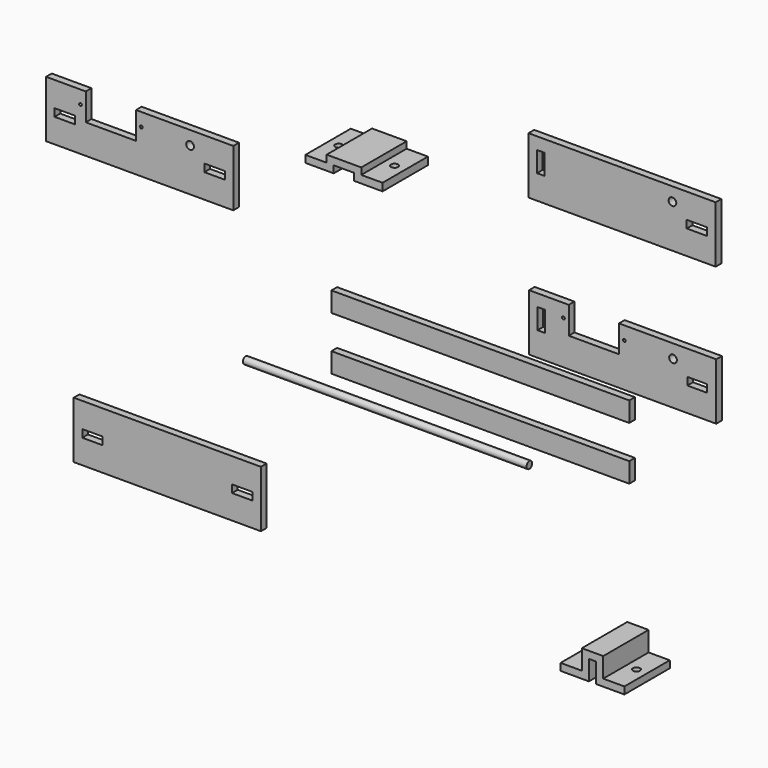
from build123d import *

# Parameters (mm, degrees)
F0_W      = 133.35
F0_H      = 8.89
F1_DEPTH  = 3.175
F2_DEPTH  = 3.175
F0_W_2    = 5.715
F0_H_2    = 3.429
F0_W_3    = 3.429
F0_H_3    = 5.715
F3_DEPTH  = 3.175
F0_W_4    = 8.89
F0_W_5    = 5.461
F4_DEPTH  = 3.175
F5_DEPTH  = 25.4
F6_R      = 1.5875
F8_DEPTH  = 97.2919927368
F0_W_6    = 9.144
F0_R      = 0.635
F0_R_2    = 1.7145
F9_DEPTH  = 3.175
F10_DEPTH = 3.175
F11_R     = 1.5875
F12_DEPTH = 127
F13_DEPTH = 25.4
F16_DEPTH = 6.5659173141


# Not quite as in the source:
# - a feature names something its author has since deleted; it is built from what else it names


with BuildPart() as f1:
    # F0 (on Front) → F1 (new body)
    with BuildSketch(Plane.XZ):
        with Locations((-66.3894339323, -18.7695804912)):
            Rectangle(F0_W, F0_H)
    extrude(amount=F1_DEPTH)


with BuildPart() as f2:
    # F0 (on Front) → F2 (new body)
    with BuildSketch(Plane.XZ):
        with Locations((-66.3894339323, -42.7141800451)):
            Rectangle(F0_W, F0_H)
    extrude(amount=F2_DEPTH)


with BuildPart() as f3:
    # F0 (on Front) → F3 (new body)
    with BuildSketch(Plane.XZ):
        Polygon((-41.0302151682, 76.3552769363), (-44.8402151682, 76.3552769363), (-44.8402151682, 50.9552769363), (38.9797848318, 50.9552769363), (38.9797848318, 76.3552769363), (35.1697848318, 76.3552769363), (19.6249848318, 76.3552769363), (9.5919848318, 76.3552769363), align=None)
        Polygon((-41.0302151682, 65.2427769363), (-41.0302151682, 70.9577769363), (-37.6012151682, 70.9577769363), (-37.6012151682, 65.2427769363), (-31.8862151682, 65.2427769363), (-31.8862151682, 61.8137769363), (-37.6012151682, 61.8137769363), (-41.0302151682, 61.8137769363), align=None, mode=Mode.SUBTRACT)
        with BuildLine():
            ThreePointArc((21.3394848318, 70.2846769363), (18.4126502554, 69.0723423599), (19.6249848318, 71.9991769363))
            ThreePointArc((19.6249848318, 71.9991769363), (20.8373194081, 71.4970115126), (21.3394848318, 70.2846769363))
        make_face(mode=Mode.SUBTRACT)
        Polygon((31.7407848318, 70.9577769363), (35.1697848318, 70.9577769363), (35.1697848318, 65.2427769363), (35.1697848318, 61.8137769363), (31.7407848318, 61.8137769363), (26.0257848318, 61.8137769363), (26.0257848318, 65.2427769363), (31.7407848318, 65.2427769363), align=None, mode=Mode.SUBTRACT)
        with Locations((-34.7437151682, 63.5282769363)):
            Rectangle(F0_W_2, F0_H_2)
        with Locations((33.4552848318, 68.1002769363)):
            Rectangle(F0_W_3, F0_H_3)
    extrude(amount=F3_DEPTH)


with BuildPart() as f4:
    # F0 (on Front) → F4 (new body)
    with BuildSketch(Plane.XZ):
        with BuildLine():
            Line((-40.7762151682, 14.5415), (-44.5862151682, 14.5415))
            Line((-44.5862151682, 14.5415), (-44.5862151682, -10.8585))
            Line((-44.5862151682, -10.8585), (-28.4685809165, -10.8585))
            Line((-28.4685809165, -10.8585), (-5.4275859147, -10.8585))
            Line((-5.4275859147, -10.8585), (35.4237848318, -10.8585))
            Line((35.4237848318, -10.8585), (39.2337848318, -10.8585))
            Line((39.2337848318, -10.8585), (39.2337848318, 14.5415))
            Line((39.2337848318, 14.5415), (9.8332848318, 14.5415))
            Line((9.8332848318, 14.5415), (-1.9396151682, 14.5415))
            Line((-1.9396151682, 14.5415), (-1.9396151682, 9.223375))
            ThreePointArc((-1.9396151682, 9.223375), (-1.4906023622, 9.0373878061), (-1.3046151682, 8.588375))
            ThreePointArc((-1.3046151682, 8.588375), (-1.3079957034, 8.5229391406), (-1.3181013153, 8.4582))
            ThreePointArc((-1.3181013153, 8.4582), (-1.9396151682, 7.953375), (-2.5611290212, 8.4582))
            Line((-2.5611290212, 8.4582), (-4.3272151682, 8.4582))
            Line((-4.3272151682, 8.4582), (-4.3272151682, 2.3749))
            Line((-4.3272151682, 2.3749), (-26.8062151682, 2.3749))
            Line((-26.8062151682, 2.3749), (-26.8062151682, 8.5979))
            Line((-26.8062151682, 8.5979), (-28.5524651682, 8.5979))
            ThreePointArc((-28.5524651682, 8.5979), (-29.6364779743, 8.1488871939), (-29.1874651682, 9.2329))
            Line((-29.1874651682, 9.2329), (-29.1874651682, 14.5415))
            Line((-29.1874651682, 14.5415), (-40.7762151682, 14.5415))
        make_face()
        Polygon((-40.7762151682, 3.429), (-40.7762151682, 9.144), (-37.3472151682, 9.144), (-37.3472151682, 3.429), (-31.8862151682, 3.429), (-31.8862151682, 0), (-37.3472151682, 0), (-40.7762151682, 0), align=None, mode=Mode.SUBTRACT)
        with Locations((30.7247848318, 1.7145)):
            Rectangle(F0_W_4, F0_H_2, mode=Mode.SUBTRACT)
        with BuildLine():
            ThreePointArc((21.5934848318, 8.4582), (19.8789848318, 6.7437), (18.1644848318, 8.4582))
            ThreePointArc((18.1644848318, 8.4582), (19.8789848318, 10.1727), (21.5934848318, 8.4582))
        make_face(mode=Mode.SUBTRACT)
        with BuildLine():
            Line((-26.8062151682, 14.5415), (-29.1874651682, 14.5415))
            Line((-29.1874651682, 14.5415), (-29.1874651682, 9.2329))
            ThreePointArc((-29.1874651682, 9.2329), (-28.7384523622, 9.0469128061), (-28.5524651682, 8.5979))
            Line((-28.5524651682, 8.5979), (-26.8062151682, 8.5979))
            Line((-26.8062151682, 8.5979), (-26.8062151682, 14.5415))
        make_face()
        with BuildLine():
            Line((-1.9396151682, 14.5415), (-4.3272151682, 14.5415))
            Line((-4.3272151682, 14.5415), (-4.3272151682, 8.588375))
            Line((-4.3272151682, 8.588375), (-4.3272151682, 8.4582))
            Line((-4.3272151682, 8.4582), (-2.5611290212, 8.4582))
            ThreePointArc((-2.5611290212, 8.4582), (-2.4325077148, 8.9887272668), (-1.9396151682, 9.223375))
            Line((-1.9396151682, 9.223375), (-1.9396151682, 14.5415))
        make_face()
        with Locations((-34.6167151682, 1.7145)):
            Rectangle(F0_W_5, F0_H_2)
    extrude(amount=F4_DEPTH)


with BuildPart() as f5:
    # F0 (on Front) → F5 (new body)
    with BuildSketch(Plane.XZ):
        Polygon((-101.9350041685, 53.3056003809), (-117.4290041685, 53.3056003809), (-117.4290041685, 50.1318126917), (-126.9540041685, 50.1318126917), (-126.9540041685, 46.9556003809), (-114.2540041685, 46.9556003809), (-114.2540041685, 50.1306003809), (-105.1100041685, 50.1306003809), (-105.1100041685, 46.9556003809), (-92.4100041685, 46.9556003809), (-92.4100041685, 50.3586865962), (-101.9350041685, 50.3586865962), align=None)
    extrude(amount=F5_DEPTH)

    # F7 (on face) + F6 (on face) → F8 (cut, through all)
    with BuildSketch(Plane.XY.offset(50.1318126917)):
        with BuildLine():
            ThreePointArc((-120.5913041685, -12.7), (-122.1788041685, -11.1125), (-123.7663041685, -12.7))
            ThreePointArc((-123.7663041685, -12.7), (-122.1788041685, -14.2875), (-120.5913041685, -12.7))
        make_face()
    with BuildSketch(Plane.XY.offset(50.3586865962)):
        with Locations((-97.1725041685, -12.7)):
            Circle(F6_R)
    extrude(amount=-F8_DEPTH, mode=Mode.SUBTRACT)


with BuildPart() as f9:
    # F0 (on Front) → F9 (new body)
    with BuildSketch(Plane.XZ):
        Polygon((-257.0258561993, 28.3309499077), (-260.8358561993, 28.3309499077), (-260.8358561993, 22.2349499077), (-260.8358561993, 2.9309499077), (-177.0158561993, 2.9309499077), (-177.0158561993, 28.3309499077), (-180.8258561993, 28.3309499077), (-206.4036561993, 28.3309499077), (-220.5768561993, 28.3309499077), (-220.5768561993, 16.1643499077), (-243.0558561993, 16.1643499077), (-243.0558561993, 28.3309499077), align=None)
        with Locations((-252.4538561993, 15.4912499077)):
            Rectangle(F0_W_6, F0_H_2, mode=Mode.SUBTRACT)
        with Locations((-245.4434561993, 22.3873499077)):
            Circle(F0_R, mode=Mode.SUBTRACT)
        with Locations((-218.1892561993, 22.3873499077)):
            Circle(F0_R, mode=Mode.SUBTRACT)
        with Locations((-196.3706561993, 22.2349499077)):
            Circle(F0_R_2, mode=Mode.SUBTRACT)
        with Locations((-185.3978561993, 15.4912499077)):
            Rectangle(F0_W_6, F0_H_2, mode=Mode.SUBTRACT)
    extrude(amount=F9_DEPTH)


with BuildPart() as f10:
    # F0 (on Front) → F10 (new body)
    with BuildSketch(Plane.XZ):
        Polygon((-244.6372990036, -94.1294633508), (-248.4472990036, -94.1294633508), (-248.4472990036, -119.5294633508), (-164.6272990036, -119.5294633508), (-164.6272990036, -94.1294633508), (-168.4372990036, -94.1294633508), align=None)
        with Locations((-240.0652990036, -106.9691633508)):
            Rectangle(F0_W_6, F0_H_2, mode=Mode.SUBTRACT)
        with Locations((-173.0092990036, -106.9691633508)):
            Rectangle(F0_W_6, F0_H_2, mode=Mode.SUBTRACT)
    extrude(amount=F10_DEPTH)


with BuildPart() as f12:
    # F11 (on Right) → F12 (new body)
    with BuildSketch(Plane.YZ):
        with Locations((-58.7386116385, -17.2708369792)):
            Circle(F11_R)
    extrude(amount=-F12_DEPTH)


with BuildPart() as f13:
    # F0 (on Front) → F13 (new body)
    with BuildSketch(Plane.XZ):
        Polygon((6.4046707157, -104.0745460367), (-3.175, -104.0745460367), (-3.175, -112.9645460367), (-12.7, -112.9645460367), (-12.7, -116.1395460367), (0, -116.1395460367), (0, -107.2495460367), (3.175, -107.2495460367), (3.175, -116.1395460367), (15.875, -116.1395460367), (15.875, -112.9650167625), (6.4046707157, -112.9650167625), align=None)
    extrude(amount=F13_DEPTH)

    # F14 (on face) + F15 (on face) → F16 (cut, through all)
    with BuildSketch(Plane.XY.offset(-112.9645460367)):
        with BuildLine():
            Line((-7.9375, -11.1125), (-7.9375, -12.7))
            Line((-7.9375, -12.7), (-7.9375, -14.2875))
            ThreePointArc((-7.9375, -14.2875), (-6.8149679849, -13.8225320151), (-6.35, -12.7))
            ThreePointArc((-6.35, -12.7), (-6.8149679849, -11.5774679849), (-7.9375, -11.1125))
        make_face()
        with BuildLine():
            Line((-7.9375, -12.7), (-9.525, -12.7))
            ThreePointArc((-9.525, -12.7), (-9.0600320151, -13.8225320151), (-7.9375, -14.2875))
            Line((-7.9375, -14.2875), (-7.9375, -12.7))
        make_face()
        with BuildLine():
            ThreePointArc((-7.9375, -11.1125), (-9.0600320151, -11.5774679849), (-9.525, -12.7))
            Line((-9.525, -12.7), (-7.9375, -12.7))
            Line((-7.9375, -12.7), (-7.9375, -11.1125))
        make_face()
    with BuildSketch(Plane.XY.offset(-112.9650167625)):
        with BuildLine():
            ThreePointArc((12.7273353579, -12.7), (11.1398353579, -11.1125), (9.5523353579, -12.7))
            ThreePointArc((9.5523353579, -12.7), (11.1398353579, -14.2875), (12.7273353579, -12.7))
        make_face()
    extrude(amount=-F16_DEPTH, mode=Mode.SUBTRACT)


solid = Compound([f1.part, f2.part, f3.part, f4.part, f5.part, f9.part, f10.part, f12.part, f13.part])
